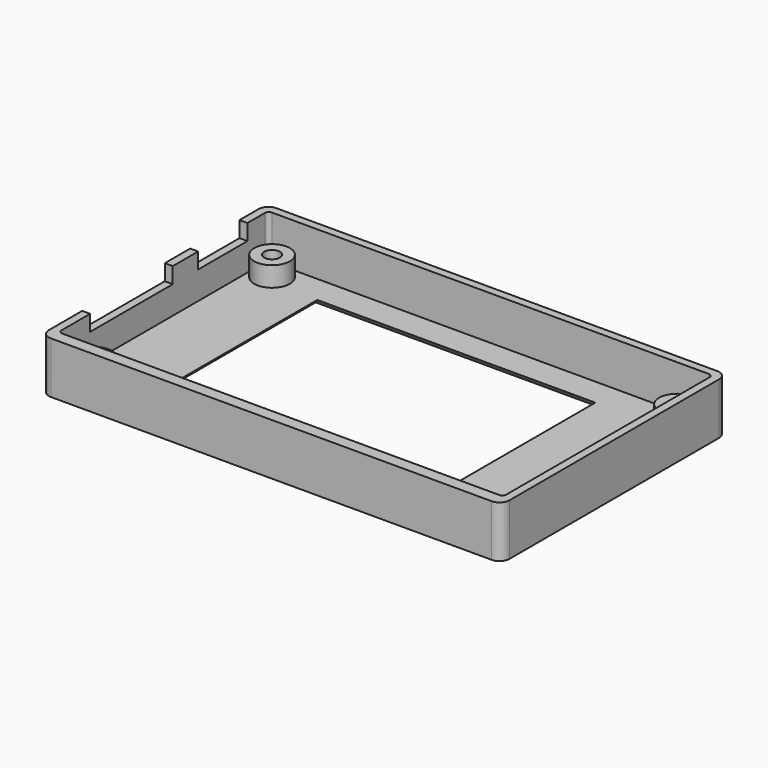
from build123d import *

# Parameters (mm, degrees)
F0_W      = 116
F0_H      = 71
F0_W_2    = 70
F0_H_2    = 53
F1_DEPTH  = 2
F2_W      = 116
F2_H      = 71
F2_W_2    = 112
F2_H_2    = 66
F3_DEPTH  = 11
F4_R      = 2.5
F5_R      = 1
F6_R      = 4.5
F6_R_2    = 2
F7_DEPTH  = 5
F8_SIZE   = 1.99999
F9_W      = 15.5
F9_H      = 7.5
F9_W_2    = 26
F9_H_2    = 4
F10_DEPTH = 25
F11_DEPTH = 25


# Not quite as in the source:
# - a fillet or chamfer is up to 0.001 mm smaller than in the source, because OpenCascade refuses the exact size


with BuildPart() as f1:
    # F0 (on Top) → F1 (new body)
    with BuildSketch(Plane.XY):
        with Locations((58, 35.5)):
            Rectangle(F0_W, F0_H)
        with Locations((55, 35.5)):
            Rectangle(F0_W_2, F0_H_2, mode=Mode.SUBTRACT)
    extrude(amount=F1_DEPTH)

    # F2 (on face) → F3 (join)
    with BuildSketch(Plane.XY.offset(2)):
        with Locations((58, 35.5)):
            Rectangle(F2_W, F2_H)
        with Locations((58, 36)):
            Rectangle(F2_W_2, F2_H_2, mode=Mode.SUBTRACT)
    extrude(amount=F3_DEPTH)

    # F4
    f4_edges = [f1.edges().sort_by_distance(p)[0] for p in [
        (0, 0, 6.5),
        (116, 0, 6.5),
        (0, 71, 6.5),
        (116, 71, 6.5),
    ]]
    fillet(f4_edges, radius=F4_R)

    # F5
    f5_edges = [f1.edges().sort_by_distance(p)[0] for p in [
        (114, 3, 7.5),
        (2, 3, 7.5),
        (2, 69, 7.5),
        (114, 69, 7.5),
    ]]
    fillet(f5_edges, radius=F5_R)

    # F6 (on face) → F7 (join)
    with BuildSketch(Plane.XY.offset(2)):
        with Locations((7, 64)):
            Circle(F6_R)
        with Locations((7, 64)):
            Circle(F6_R_2, mode=Mode.SUBTRACT)
        with Locations((7, 8)):
            Circle(F6_R)
        with Locations((7, 8)):
            Circle(F6_R_2, mode=Mode.SUBTRACT)
        with Locations((109, 8)):
            Circle(F6_R)
        with Locations((109, 8)):
            Circle(F6_R_2, mode=Mode.SUBTRACT)
        with Locations((109, 64)):
            Circle(F6_R)
        with Locations((109, 64)):
            Circle(F6_R_2, mode=Mode.SUBTRACT)
    extrude(amount=F7_DEPTH)

    # F8 (size 2 in the source; OpenCascade refuses exactly that, so slightly less here)
    f8_edges = [f1.edges().sort_by_distance(p)[0] for p in [
        (90, 35.5, 0),
        (55, 9, 0),
        (20, 35.5, 0),
        (55, 62, 0),
    ]]
    chamfer(f8_edges, length=F8_SIZE)

    # F9 (on face) → F10 (cut)
    with BuildSketch(Plane(origin=(0, 0, 0), x_dir=(0, -1, 0), z_dir=(-1, 0, 0))):
        with Locations((-54.75, 12.75)):
            Rectangle(F9_W, F9_H)
        with Locations((-26, 11)):
            Rectangle(F9_W_2, F9_H_2)
    extrude(amount=-F10_DEPTH, mode=Mode.SUBTRACT)

    # F11 (cut): faces of the model
    f11_faces = [f1.faces().sort_by_distance(p)[0] for p in [
        (7, 8, 2),
        (7, 64, 2),
        (109, 8, 2),
        (109, 64, 2),
    ]]
    extrude(f11_faces, amount=-F11_DEPTH, mode=Mode.SUBTRACT)


solid = f1.part
